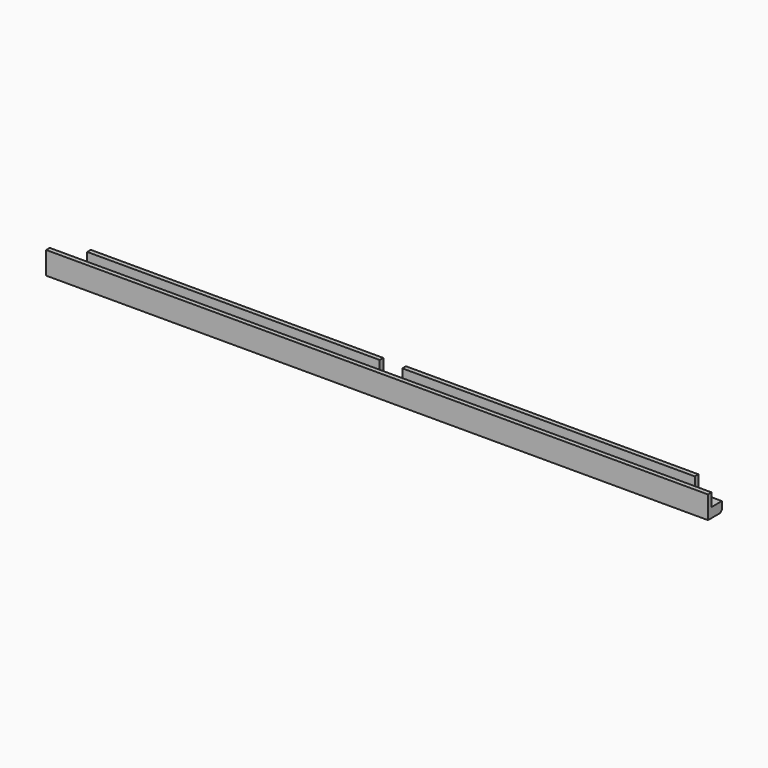
from build123d import *

# Parameters (mm, degrees)
F1_DEPTH = 4.3
F0_W     = 129.25
F0_H     = 2
F0_W_2   = 146.25
F2_DEPTH = 10
F3_SIZE  = 3


# Not quite as in the source:
# - a feature names something its author has since deleted; it is built from what else it names


with BuildPart() as f1:
    # F0 (on Top) → F1 (new body)
    with BuildSketch(Plane.XY):
        Polygon((0, 2.85), (0, -2.85), (146.25, -2.85), (146.25, 2.85), (139.25, 2.85), (134.25, 2.85), (5, 2.85), align=None)
        Polygon((-139.25, 2.85), (-146.25, 2.85), (-146.25, -2.85), (0, -2.85), (0, 2.85), (-5, 2.85), (-134.25, 2.85), align=None)
    extrude(amount=F1_DEPTH)

    # F0 (on Top) → F2 (join)
    with BuildSketch(Plane.XY):
        with Locations((69.625, 3.85)):
            Rectangle(F0_W, F0_H)
        with Locations((73.125, -3.85)):
            Rectangle(F0_W_2, F0_H)
        with Locations((-73.125, -3.85)):
            Rectangle(F0_W_2, F0_H)
        with Locations((-69.625, 3.85)):
            Rectangle(F0_W, F0_H)
    extrude(amount=F2_DEPTH)

    # F3
    f3_edges = [f1.edges().sort_by_distance(p)[0] for p in [
        (69.625, 4.85, 0),
    ]]
    chamfer(f3_edges, length=F3_SIZE)


solid = f1.part
